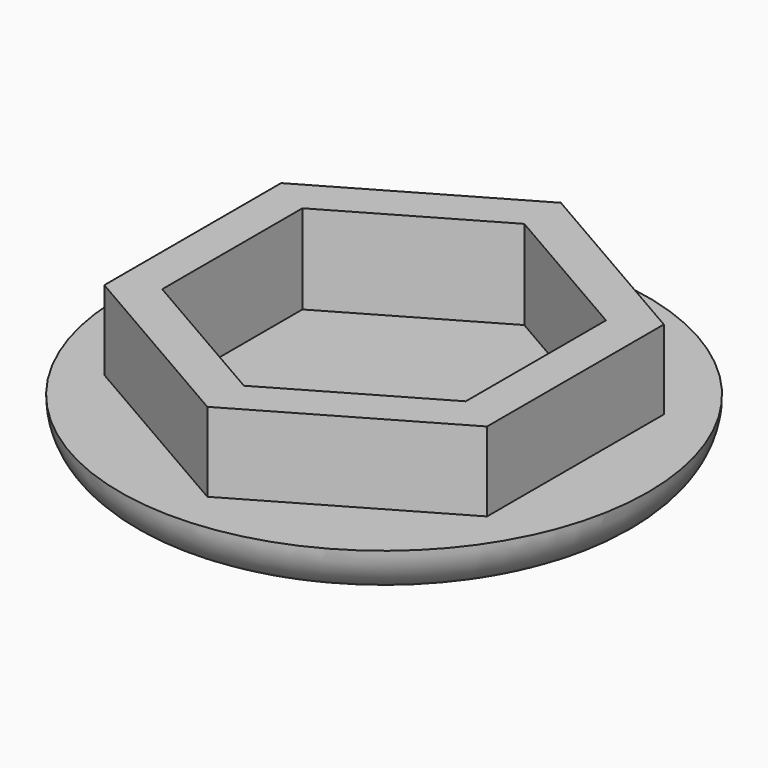
from build123d import *

# Parameters (mm, degrees)
F0_R     = 8
F1_DEPTH = 1.5
F3_DEPTH = 2.4
F4_T     = -1.2
F5_R     = 1.49999


# Not quite as in the source:
# - a fillet or chamfer is up to 0.001 mm smaller than in the source, because OpenCascade refuses the exact size


with BuildPart() as f1:
    # F0 (on Top) → F1 (new body)
    with BuildSketch(Plane.XY):
        Circle(F0_R)
    extrude(amount=F1_DEPTH)

    # F2 (on face) → F3 (join)
    with BuildSketch(Plane.XY.offset(1.5)):
        Polygon((5.8, -3.3486315613), (5.8, 3.3486315613), (0, 6.6972631226), (-5.8, 3.3486315613), (-5.8, -3.3486315613), (0, -6.6972631226), align=None)
    extrude(amount=F3_DEPTH)

    # F4
    f4_openings = [f1.faces().sort_by_distance(p)[0] for p in [
        (0, 0, 3.9),
    ]]
    offset(amount=F4_T, openings=f4_openings, kind=Kind.INTERSECTION)

    # F5 (radius 1.5 in the source; OpenCascade refuses exactly that, so slightly less here)
    f5_edges = [f1.edges().sort_by_distance(p)[0] for p in [
        (-8, 0, 0),
    ]]
    fillet(f5_edges, radius=F5_R)


solid = f1.part
